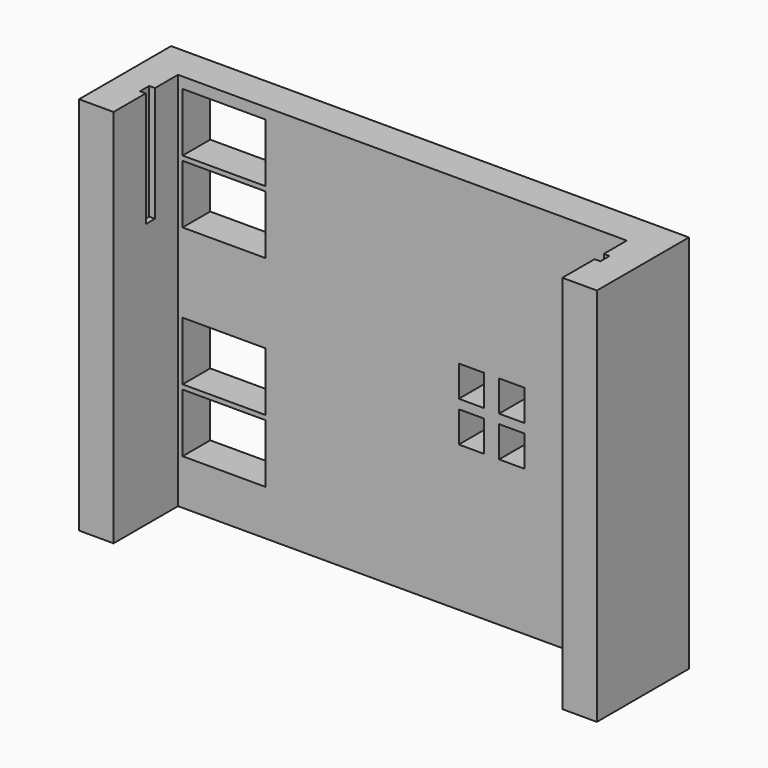
from build123d import *

# Parameters (mm, degrees)
F0_W          = 114.3
F0_H          = 83.82
F1_DEPTH      = 7.62
F2_W          = 7.62
F2_H          = 83.82
F3_DEPTH      = 17.78
F4_W          = 1.27
F4_H          = 2.54
F5_DEPTH      = 25.4
F6_W          = 18.288
F6_H          = 12.954
F7_DEPTH      = 25.4
F8_W          = 5.588
F8_H          = 6.858
F9_DEPTH      = 25.4
F10_TEXT_SIZE = 1.3926552059
F11_DEPTH     = 0.254
F12_TEXT_SIZE = 1.3296253885
F13_DEPTH     = 0.254
F14_TEXT_SIZE = 1.4177568463
F15_DEPTH     = 0.254
F16_TEXT_SIZE = 1.3516025825
F17_DEPTH     = 0.254
F18_R         = 1.27
F19_DEPTH     = 0.508


# Not quite as in the source:
# - Text() gives the source's letters only with a copy of the font that has no kerning and outlines rounded to 1/6400 em; it was checked with that copy


with BuildPart() as f1:
    # F0 (on Front) → F1 (new body)
    with BuildSketch(Plane.XZ):
        Rectangle(F0_W, F0_H)
    extrude(amount=F1_DEPTH)

    # F2 (on face) → F3 (join)
    with BuildSketch(Plane.XZ.offset(7.62)):
        with Locations((-53.34, 0)):
            Rectangle(F2_W, F2_H)
        with Locations((53.34, 0)):
            Rectangle(F2_W, F2_H)
    extrude(amount=F3_DEPTH)

    # F4 (on face) → F5 (cut)
    with BuildSketch(Plane.XY.offset(41.91)):
        with Locations((-50.165, -15.24)):
            Rectangle(F4_W, F4_H)
        with Locations((50.165, -15.24)):
            Rectangle(F4_W, F4_H)
    extrude(amount=-F5_DEPTH, mode=Mode.SUBTRACT)

    # F6 (on face) → F7 (cut)
    with BuildSketch(Plane.XZ.offset(7.62)):
        with Locations((-39.37, 33.02)):
            Rectangle(F6_W, F6_H)
        with Locations((-39.37, 19.05)):
            Rectangle(F6_W, F6_H)
        with Locations((-39.37, -11.43)):
            Rectangle(F6_W, F6_H)
        with Locations((-39.37, -25.4)):
            Rectangle(F6_W, F6_H)
    extrude(amount=-F7_DEPTH, mode=Mode.SUBTRACT)

    # F8 (on face) → F9 (cut)
    with BuildSketch(Plane(origin=(0, 0, 0), x_dir=(-1, 0, 0), z_dir=(0, 1, 0))):
        with Locations((-24.13, 2.54)):
            Rectangle(F8_W, F8_H)
        with Locations((-15.24, 2.54)):
            Rectangle(F8_W, F8_H)
        with Locations((-24.13, -6.35)):
            Rectangle(F8_W, F8_H)
        with Locations((-15.24, -6.35)):
            Rectangle(F8_W, F8_H)
    extrude(amount=-F9_DEPTH, mode=Mode.SUBTRACT)

    # F10 (on face) → F11 (join)
    with BuildSketch(Plane(origin=(0, 0, 0), x_dir=(-1, 0, 0), z_dir=(0, 1, 0))):
        with Locations((-17.0419326293, 6.2196567026)):
            Text('hours', F10_TEXT_SIZE, font='Open Sans', text_align=(TextAlign.LEFT, TextAlign.BOTTOM))
    extrude(amount=F11_DEPTH)

    # F12 (on face) → F13 (join)
    with BuildSketch(Plane(origin=(0, 0, 0), x_dir=(-1, 0, 0), z_dir=(0, 1, 0))):
        with Locations((-26.6051976002, 6.1851104686)):
            Text('minutes', F12_TEXT_SIZE, font='Open Sans', text_align=(TextAlign.LEFT, TextAlign.BOTTOM))
    extrude(amount=F13_DEPTH)

    # F14 (on face) → F15 (join)
    with BuildSketch(Plane(origin=(0, 0, 0), x_dir=(-1, 0, 0), z_dir=(0, 1, 0))):
        with Locations((-26.035, -11.0719978788)):
            Text('alarm', F14_TEXT_SIZE, font='Open Sans', text_align=(TextAlign.LEFT, TextAlign.BOTTOM))
    extrude(amount=F15_DEPTH)

    # F16 (on face) → F17 (join)
    with BuildSketch(Plane(origin=(0, 0, 0), x_dir=(-1, 0, 0), z_dir=(0, 1, 0))):
        with Locations((-16.8540035526, -11.0763115808)):
            Text('clock', F16_TEXT_SIZE, font='Open Sans', text_align=(TextAlign.LEFT, TextAlign.BOTTOM))
    extrude(amount=F17_DEPTH)

    # F18 (on face) → F19 (join)
    with BuildSketch(Plane(origin=(0, 0, 0), x_dir=(-1, 0, 0), z_dir=(0, 1, 0))):
        with Locations((42.418, 3.3993879333)):
            Circle(F18_R)
        with Locations((36.068, 3.4036)):
            Circle(F18_R)
    extrude(amount=F19_DEPTH)


solid = f1.part
